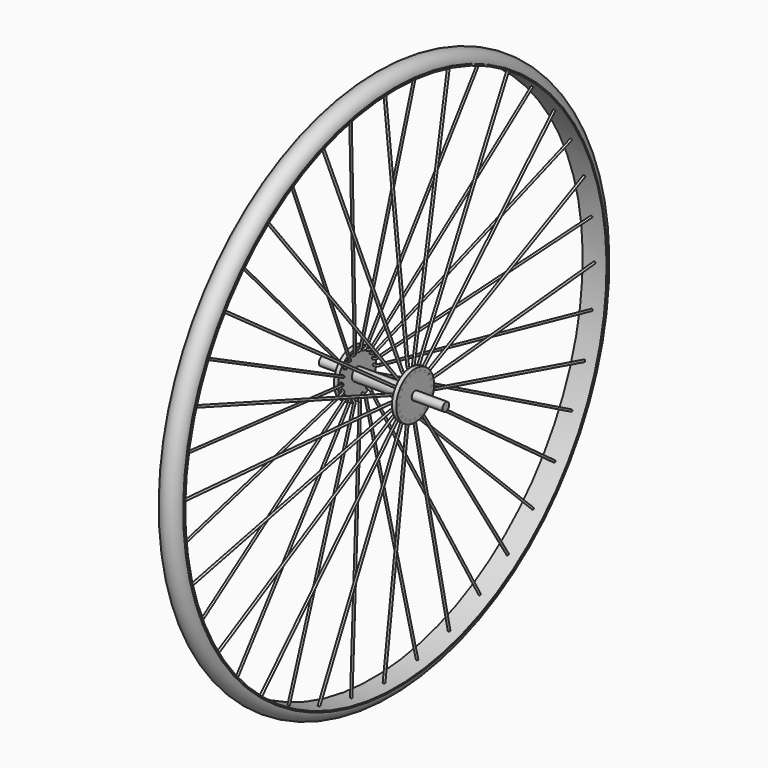
from build123d import *

# Parameters (mm, degrees)
F3_R      = 1
F4_DEPTH  = 58.001
F16_R     = 0.99
F18_COUNT = 20
F21_R     = 0.9
F26_COUNT = 20
F27_R     = 4
F28_DEPTH = 58.001
F29_R     = 3.9
F30_DEPTH = 57.5


# Not quite as in the source:
# - a feature names something its author has since deleted; it is built from what else it names


with BuildPart() as f2:
    # F1 (on Front) → F2 (revolve)
    with BuildSketch(Plane.XZ):
        Polygon((25, 6), (0, 6), (-25, 6), (-25, 22), (-29, 22), (-29, 0), (29, 0), (29, 22), (25, 22), align=None)
    revolve(axis=Axis((2.9746498913, 0, 0), (1, 0, 0)))

    # F3 (on face) → F4 (cut, through all)
    with BuildSketch(Plane.YZ.offset(29)):
        with Locations((0, 19)):
            Circle(F3_R)
        with Locations((-5.8713228931, 18.0700738096)):
            Circle(F3_R)
        with Locations((-11.1679197936, 15.3713228931)):
            Circle(F3_R)
        with Locations((-15.3713228931, 11.1679197936)):
            Circle(F3_R)
        with Locations((-18.0700738096, 5.8713228931)):
            Circle(F3_R)
        with Locations((-19, 0)):
            Circle(F3_R)
        with Locations((-18.0700738096, -5.8713228931)):
            Circle(F3_R)
        with Locations((-15.3713228931, -11.1679197936)):
            Circle(F3_R)
        with Locations((-11.1679197936, -15.3713228931)):
            Circle(F3_R)
        with Locations((-5.8713228931, -18.0700738096)):
            Circle(F3_R)
        with Locations((0, -19)):
            Circle(F3_R)
        with Locations((5.8713228931, -18.0700738096)):
            Circle(F3_R)
        with Locations((11.1679197936, -15.3713228931)):
            Circle(F3_R)
        with Locations((15.3713228931, -11.1679197936)):
            Circle(F3_R)
        with Locations((18.0700738096, -5.8713228931)):
            Circle(F3_R)
        with Locations((19, 0)):
            Circle(F3_R)
        with Locations((11.1679197936, 15.3713228931)):
            Circle(F3_R)
        with Locations((15.3713228931, 11.1679197936)):
            Circle(F3_R)
        with Locations((18.0700738096, 5.8713228931)):
            Circle(F3_R)
        with Locations((5.8713228931, 18.0700738096)):
            Circle(F3_R)
    extrude(amount=-F4_DEPTH, mode=Mode.SUBTRACT)

    # F27 (on face) → F28 (cut, through all)
    with BuildSketch(Plane.YZ.offset(29)):
        Circle(F27_R)
    extrude(amount=-F28_DEPTH, mode=Mode.SUBTRACT)


with BuildPart() as f6:
    # F5 (on Front) → F6 (revolve)
    with BuildSketch(Plane.XZ):
        with BuildLine():
            Line((-10, 246), (10, 246))
            ThreePointArc((10, 246), (0, 256), (-10, 246))
        make_face()
    revolve(axis=Axis((2.9746498913, 0, 0), (1, 0, 0)))


with BuildPart() as f8:
    # F7 (on Front) → F8 (revolve)
    with BuildSketch(Plane.XZ):
        Polygon((10.1, 246.1), (10.1, 245.9), (0, 245.9), (-10.1, 245.9), (-10.1, 246.1), (-11.1, 246.1), (-11.1, 244.9), (0, 244.9), (11.1, 244.9), (11.1, 246.1), align=None)
    revolve(axis=Axis((2.9746498913, 0, 0), (1, 0, 0)))


with BuildPart() as f17:
    # F17: sweep along a path in F11
    with BuildLine(Plane.XZ) as f17_path:
        Line((29, 19), (25, 19))
        ThreePointArc((25, 19), (22.9854765706, 19.7770075681), (22.0144864417, 21.7055364319))
        Line((22.0144864417, 21.7055364319), (0, 244.9064850807))
    # F16 (on line) → F17 (sweep)
    with BuildSketch(Plane.YZ.offset(29)):
        with Locations((0, 19)):
            Circle(F16_R)
    sweep(path=f17_path.line)


with BuildPart() as f18_1:
    # F18: instance of F17
    add(f17.part.rotate(Axis((2.9746498913, 0, 0), (1, 0, 0)), 1 * 360 / F18_COUNT))


with BuildPart() as f18_2:
    # F18: instance of F17
    add(f17.part.rotate(Axis((2.9746498913, 0, 0), (1, 0, 0)), 2 * 360 / F18_COUNT))


with BuildPart() as f18_3:
    # F18: instance of F17
    add(f17.part.rotate(Axis((2.9746498913, 0, 0), (1, 0, 0)), 3 * 360 / F18_COUNT))


with BuildPart() as f18_4:
    # F18: instance of F17
    add(f17.part.rotate(Axis((2.9746498913, 0, 0), (1, 0, 0)), 4 * 360 / F18_COUNT))


with BuildPart() as f18_5:
    # F18: instance of F17
    add(f17.part.rotate(Axis((2.9746498913, 0, 0), (1, 0, 0)), 5 * 360 / F18_COUNT))


with BuildPart() as f18_6:
    # F18: instance of F17
    add(f17.part.rotate(Axis((2.9746498913, 0, 0), (1, 0, 0)), 6 * 360 / F18_COUNT))


with BuildPart() as f18_7:
    # F18: instance of F17
    add(f17.part.rotate(Axis((2.9746498913, 0, 0), (1, 0, 0)), 7 * 360 / F18_COUNT))


with BuildPart() as f18_8:
    # F18: instance of F17
    add(f17.part.rotate(Axis((2.9746498913, 0, 0), (1, 0, 0)), 8 * 360 / F18_COUNT))


with BuildPart() as f18_9:
    # F18: instance of F17
    add(f17.part.rotate(Axis((2.9746498913, 0, 0), (1, 0, 0)), 9 * 360 / F18_COUNT))


with BuildPart() as f18_10:
    # F18: instance of F17
    add(f17.part.rotate(Axis((2.9746498913, 0, 0), (1, 0, 0)), 10 * 360 / F18_COUNT))


with BuildPart() as f18_11:
    # F18: instance of F17
    add(f17.part.rotate(Axis((2.9746498913, 0, 0), (1, 0, 0)), 11 * 360 / F18_COUNT))


with BuildPart() as f18_12:
    # F18: instance of F17
    add(f17.part.rotate(Axis((2.9746498913, 0, 0), (1, 0, 0)), 12 * 360 / F18_COUNT))


with BuildPart() as f18_13:
    # F18: instance of F17
    add(f17.part.rotate(Axis((2.9746498913, 0, 0), (1, 0, 0)), 13 * 360 / F18_COUNT))


with BuildPart() as f18_14:
    # F18: instance of F17
    add(f17.part.rotate(Axis((2.9746498913, 0, 0), (1, 0, 0)), 14 * 360 / F18_COUNT))


with BuildPart() as f18_15:
    # F18: instance of F17
    add(f17.part.rotate(Axis((2.9746498913, 0, 0), (1, 0, 0)), 15 * 360 / F18_COUNT))


with BuildPart() as f18_16:
    # F18: instance of F17
    add(f17.part.rotate(Axis((2.9746498913, 0, 0), (1, 0, 0)), 16 * 360 / F18_COUNT))


with BuildPart() as f18_17:
    # F18: instance of F17
    add(f17.part.rotate(Axis((2.9746498913, 0, 0), (1, 0, 0)), 17 * 360 / F18_COUNT))


with BuildPart() as f18_18:
    # F18: instance of F17
    add(f17.part.rotate(Axis((2.9746498913, 0, 0), (1, 0, 0)), 18 * 360 / F18_COUNT))


with BuildPart() as f18_19:
    # F18: instance of F17
    add(f17.part.rotate(Axis((2.9746498913, 0, 0), (1, 0, 0)), 19 * 360 / F18_COUNT))


with BuildPart() as f25:
    # F25: sweep along a path in F24
    with BuildLine(Plane(origin=(0, -3.1377191364, -0.4628140463), x_dir=(1, 0, 0), z_dir=(0, -0.9892961958, -0.1459213382))) as f25_path:
        Line((-29, 18.7334065717), (-25, 18.7334065717))
        ThreePointArc((-25, 18.7334065717), (-22.9840036139, 19.511749854), (-22.014098724, 21.4429008576))
        Line((-22.014098724, 21.4429008576), (0, 247.7101385593))
    # F21 (on face) → F25 (sweep)
    with BuildSketch(Plane(origin=(-29, 0, 0), x_dir=(0, -1, 0), z_dir=(-1, 0, 0))):
        with Locations((5.8713228931, 18.0700738096)):
            Circle(F21_R)
    sweep(path=f25_path.line)


with BuildPart() as f26_1:
    # F26: instance of F25
    add(f25.part.rotate(Axis((2.9746498913, 0, 0), (1, 0, 0)), 1 * 360 / F26_COUNT))


with BuildPart() as f26_2:
    # F26: instance of F25
    add(f25.part.rotate(Axis((2.9746498913, 0, 0), (1, 0, 0)), 2 * 360 / F26_COUNT))


with BuildPart() as f26_3:
    # F26: instance of F25
    add(f25.part.rotate(Axis((2.9746498913, 0, 0), (1, 0, 0)), 3 * 360 / F26_COUNT))


with BuildPart() as f26_4:
    # F26: instance of F25
    add(f25.part.rotate(Axis((2.9746498913, 0, 0), (1, 0, 0)), 4 * 360 / F26_COUNT))


with BuildPart() as f26_5:
    # F26: instance of F25
    add(f25.part.rotate(Axis((2.9746498913, 0, 0), (1, 0, 0)), 5 * 360 / F26_COUNT))


with BuildPart() as f26_6:
    # F26: instance of F25
    add(f25.part.rotate(Axis((2.9746498913, 0, 0), (1, 0, 0)), 6 * 360 / F26_COUNT))


with BuildPart() as f26_7:
    # F26: instance of F25
    add(f25.part.rotate(Axis((2.9746498913, 0, 0), (1, 0, 0)), 7 * 360 / F26_COUNT))


with BuildPart() as f26_8:
    # F26: instance of F25
    add(f25.part.rotate(Axis((2.9746498913, 0, 0), (1, 0, 0)), 8 * 360 / F26_COUNT))


with BuildPart() as f26_9:
    # F26: instance of F25
    add(f25.part.rotate(Axis((2.9746498913, 0, 0), (1, 0, 0)), 9 * 360 / F26_COUNT))


with BuildPart() as f26_10:
    # F26: instance of F25
    add(f25.part.rotate(Axis((2.9746498913, 0, 0), (1, 0, 0)), 10 * 360 / F26_COUNT))


with BuildPart() as f26_11:
    # F26: instance of F25
    add(f25.part.rotate(Axis((2.9746498913, 0, 0), (1, 0, 0)), 11 * 360 / F26_COUNT))


with BuildPart() as f26_12:
    # F26: instance of F25
    add(f25.part.rotate(Axis((2.9746498913, 0, 0), (1, 0, 0)), 12 * 360 / F26_COUNT))


with BuildPart() as f26_13:
    # F26: instance of F25
    add(f25.part.rotate(Axis((2.9746498913, 0, 0), (1, 0, 0)), 13 * 360 / F26_COUNT))


with BuildPart() as f26_14:
    # F26: instance of F25
    add(f25.part.rotate(Axis((2.9746498913, 0, 0), (1, 0, 0)), 14 * 360 / F26_COUNT))


with BuildPart() as f26_15:
    # F26: instance of F25
    add(f25.part.rotate(Axis((2.9746498913, 0, 0), (1, 0, 0)), 15 * 360 / F26_COUNT))


with BuildPart() as f26_16:
    # F26: instance of F25
    add(f25.part.rotate(Axis((2.9746498913, 0, 0), (1, 0, 0)), 16 * 360 / F26_COUNT))


with BuildPart() as f26_17:
    # F26: instance of F25
    add(f25.part.rotate(Axis((2.9746498913, 0, 0), (1, 0, 0)), 17 * 360 / F26_COUNT))


with BuildPart() as f26_18:
    # F26: instance of F25
    add(f25.part.rotate(Axis((2.9746498913, 0, 0), (1, 0, 0)), 18 * 360 / F26_COUNT))


with BuildPart() as f26_19:
    # F26: instance of F25
    add(f25.part.rotate(Axis((2.9746498913, 0, 0), (1, 0, 0)), 19 * 360 / F26_COUNT))


with BuildPart() as f30:
    # F29 (on Right) → F30 (new body, symmetric)
    with BuildSketch(Plane.YZ):
        Circle(F29_R)
    extrude(amount=F30_DEPTH, both=True)


solid = Compound([f2.part, f6.part, f8.part, f17.part, f18_1.part, f18_2.part, f18_3.part, f18_4.part, f18_5.part, f18_6.part, f18_7.part, f18_8.part, f18_9.part, f18_10.part, f18_11.part, f18_12.part, f18_13.part, f18_14.part, f18_15.part, f18_16.part, f18_17.part, f18_18.part, f18_19.part, f25.part, f26_1.part, f26_2.part, f26_3.part, f26_4.part, f26_5.part, f26_6.part, f26_7.part, f26_8.part, f26_9.part, f26_10.part, f26_11.part, f26_12.part, f26_13.part, f26_14.part, f26_15.part, f26_16.part, f26_17.part, f26_18.part, f26_19.part, f30.part])
